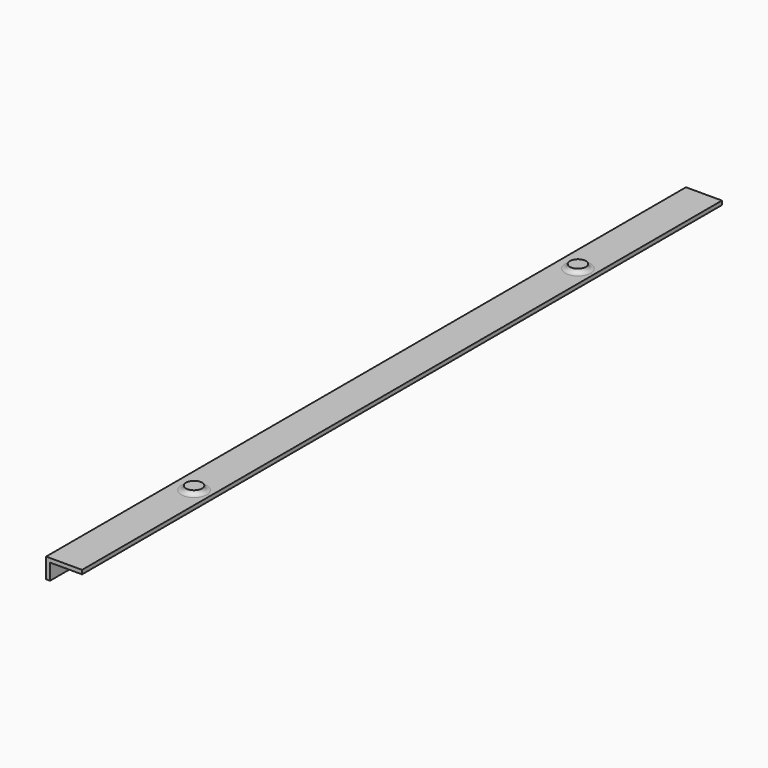
from build123d import *

# Parameters (mm, degrees)
F1_DEPTH = 635
F2_R     = 12.7
F3_DEPTH = 12.7


# Not quite as in the source:
# - a fillet or chamfer that OpenCascade refuses, or shapes differently, is made with other operations: its cross-section is extruded or revolved along the edge and cut away or added


with BuildPart() as f1:
    # F0 (on Front) → F1 (new body, symmetric)
    with BuildSketch(Plane.XZ):
        Polygon((-50.8, 0), (0, 0), (0, 6.35), (-57.15, 6.35), (-57.15, -25.4), (-50.8, -25.4), align=None)
    extrude(amount=F1_DEPTH, both=True)

    # F2 (on Top) → F3 (join)
    with BuildSketch(Plane.XY):
        with Locations((-25.4, 381)):
            Circle(F2_R)
        with Locations((-25.4, -381)):
            Circle(F2_R)
    extrude(amount=F3_DEPTH)

    # F4: fillet of radius 7.62 on 1 edges, made by hand

    # F4_s1 → F4_t2 (revolve)
    with BuildSketch(Plane.XZ.offset(-381)):
        with BuildLine():
            ThreePointArc((-5.1865786755, 6.35), (-10.1052675251, 8.1501288674), (-12.7, 12.7))
            Line((-12.7, 12.7), (-12.7, 6.35))
            Line((-12.7, 6.35), (-5.1865786755, 6.35))
        make_face()
    revolve(axis=Axis((-25.4, 381, 6.35), (0, 0, -1)))

    # F5: fillet of radius 7.62 on 1 edges, made by hand

    # F5_s1 → F5_t2 (revolve)
    with BuildSketch(Plane.XZ.offset(381)):
        with BuildLine():
            ThreePointArc((-5.1865786755, 6.35), (-10.1052675251, 8.1501288674), (-12.7, 12.7))
            Line((-12.7, 12.7), (-12.7, 6.35))
            Line((-12.7, 6.35), (-5.1865786755, 6.35))
        make_face()
    revolve(axis=Axis((-25.4, -381, 6.35), (0, 0, -1)))


solid = f1.part
